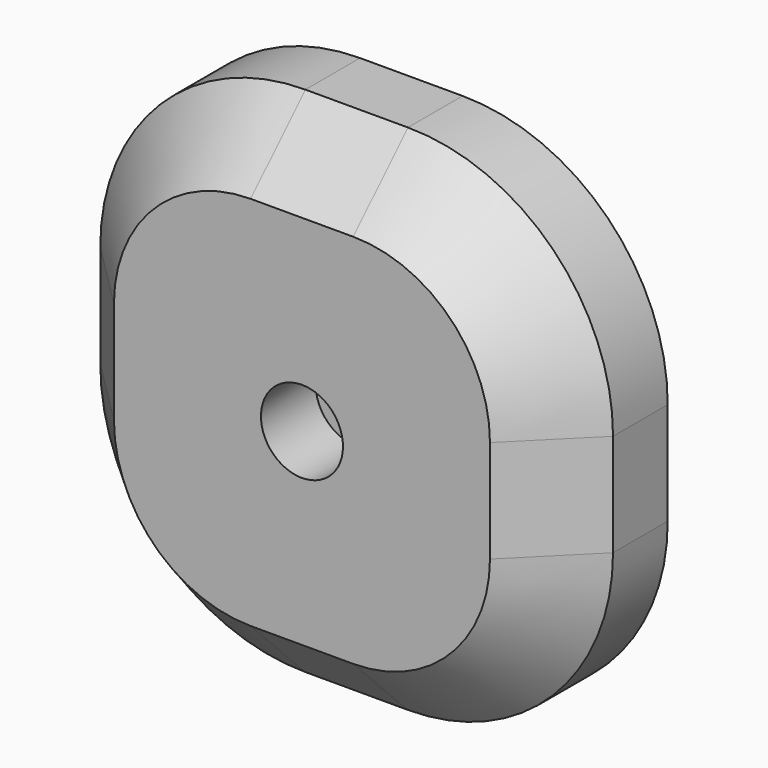
from build123d import *

# Parameters (mm, degrees)
F0_W     = 75
F0_H     = 75
F1_DEPTH = 20
F2_R     = 30
F5_SIZE  = 10
F3_R     = 6
F4_R     = 6
F6_DEPTH = 10
F7_DEPTH = 10


with BuildPart() as f1:
    # F0 (on Front) → F1 (new body)
    with BuildSketch(Plane.XZ):
        with Locations((-37.5, 37.5)):
            Rectangle(F0_W, F0_H)
    extrude(amount=F1_DEPTH)

    # F2
    f2_edges = [f1.edges().sort_by_distance(p)[0] for p in [
        (-75, -10, 0),
        (0, -10, 0),
        (0, -10, 75),
        (-75, -10, 75),
    ]]
    fillet(f2_edges, radius=F2_R)

    # F5
    f5_edges = [f1.edges().sort_by_distance(p)[0] for p in [
        (-75, -20, 37.5),
        (-37.5, -20, 0),
        (-66.213203, -20, 8.786797),
        (-8.786797, -20, 8.786797),
        (0, -20, 37.5),
        (-66.213203, -20, 66.213203),
        (-8.786797, -20, 66.213203),
        (-37.5, -20, 75),
    ]]
    chamfer(f5_edges, length=F5_SIZE)

    # F3 (on face) + F4 (on face) → F6 (cut)
    with BuildSketch(Plane.XZ.offset(20)):
        with Locations((-37.5, 37.5)):
            Circle(F3_R)
    with BuildSketch(Plane(origin=(0, 0, 0), x_dir=(-1, 0, 0), z_dir=(0, 1, 0))):
        with Locations((50, 25)):
            Circle(F4_R)
        with Locations((25, 25)):
            Circle(F4_R)
        with Locations((25, 50)):
            Circle(F4_R)
        with Locations((50, 50)):
            Circle(F4_R)
    extrude(amount=-F6_DEPTH, dir=(0, -1, 0), mode=Mode.SUBTRACT)

    # F4 (on face) → F7 (cut)
    with BuildSketch(Plane(origin=(0, 0, 0), x_dir=(-1, 0, 0), z_dir=(0, 1, 0))):
        with Locations((25, 50)):
            Circle(F4_R)
        with Locations((50, 50)):
            Circle(F4_R)
        with Locations((50, 25)):
            Circle(F4_R)
        with Locations((25, 25)):
            Circle(F4_R)
    extrude(amount=-F7_DEPTH, mode=Mode.SUBTRACT)


solid = f1.part
